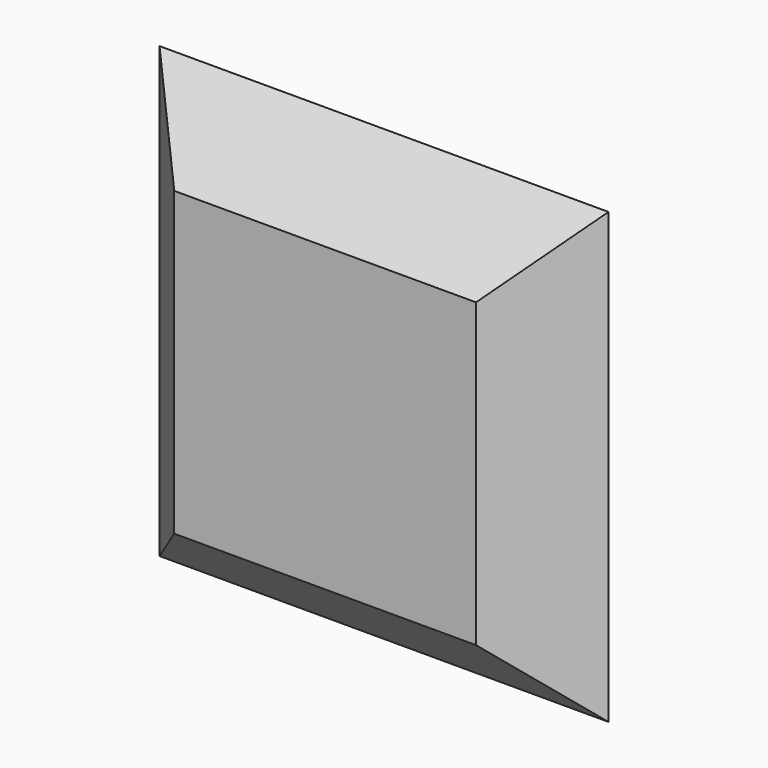
from build123d import *

# Parameters (mm, degrees)
F1_DEPTH     = 3
F2_SIZE2     = 1.49999
F2_SIZE      = 1.49999
F3_W         = 1.7351090792
F3_H         = 1.7351090792
F4_DEPTH     = 0.45
F5_T4_DEPTH  = 3.4702181583
F5_T9_DEPTH  = 3.4702181583
F5_T14_DEPTH = 3.4702181583
F5_T19_DEPTH = 3.4702181583
F6_T1_DEPTH  = 16.5056825173
F6_T3_DEPTH  = 16.5056825173


# Not quite as in the source:
# - a fillet or chamfer that OpenCascade refuses, or shapes differently, is made with other operations: its cross-section is extruded or revolved along the edge and cut away or added
# - a fillet or chamfer is up to 0.001 mm smaller than in the source, because OpenCascade refuses the exact size


with BuildPart() as f1:
    # F0 (on Front) → F1 (new body)
    with BuildSketch(Plane.XZ):
        Polygon((4.575161729, 4.575161729), (0, 4.575161729), (-4.575161729, 4.575161729), (-4.575161729, 0), (-4.575161729, -4.575161729), (0, -4.575161729), (4.575161729, -4.575161729), (4.575161729, 0), align=None)
    extrude(amount=F1_DEPTH)

    # F2 (size 1.5 and 1.5 in the source; OpenCascade refuses exactly that, so slightly less here)
    f2_edges = [f1.edges().sort_by_distance(p)[0] for p in [
        (0, -3, 4.575162),
        (-4.575162, -3, 0),
        (0, -3, -4.575162),
        (4.575162, -3, 0),
        (0, 0, 4.575162),
        (-4.575162, 0, 0),
        (0, 0, -4.575162),
        (4.575162, 0, 0),
    ]]
    chamfer(f2_edges, length=F2_SIZE, length2=F2_SIZE2)

    # F3 (on face) → F4 (cut)
    with BuildSketch(Plane(origin=(0, 0, 0), x_dir=(-1, 0, 0), z_dir=(0, 1, 0))):
        Polygon((0, 1.7351090792), (0, 0), (-1.7351090792, 0), (-1.7351090792, -1.7351090792), (0, -1.7351090792), (1.7351090792, -1.7351090792), (1.7351090792, 0), (1.7351090792, 1.7351090792), align=None)
        with Locations((-0.8675545396, 0.8675545396)):
            Rectangle(F3_W, F3_H)
    extrude(amount=-F4_DEPTH, mode=Mode.SUBTRACT)

    # F5: chamfer of 0.6 on 4 edges, made by hand


with BuildPart() as f5_tool2:
    # F5_s3 → F5_t4 (new body)
    with BuildSketch(Plane.YZ.offset(-1.7351090792)):
        Polygon((0.15, 1.7351090792), (-0.45, 1.1351090792), (-0.45, 1.7351090792), align=None)
    extrude(amount=F5_T4_DEPTH)

    split(bisect_by=Plane.XZ, keep=Keep.TOP)


with BuildPart() as f1_1:
    add(f1.part)

    # F5_t1: union F5_tool2
    add(f5_tool2.part)


with BuildPart() as f5_tool7:
    # F5_s8 → F5_t9 (new body)
    with BuildSketch(Plane.XY.offset(1.7351090792)):
        Polygon((1.7351090792, 0.15), (1.1351090792, -0.45), (1.7351090792, -0.45), align=None)
    extrude(amount=-F5_T9_DEPTH)

    split(bisect_by=Plane.XZ, keep=Keep.TOP)


with BuildPart() as f1_2:
    add(f1_1.part)

    # F5_t6: union F5_tool7
    add(f5_tool7.part)


with BuildPart() as f5_tool12:
    # F5_s13 → F5_t14 (new body)
    with BuildSketch(Plane.YZ.offset(1.7351090792)):
        Polygon((0.15, -1.7351090792), (-0.45, -1.1351090792), (-0.45, -1.7351090792), align=None)
    extrude(amount=-F5_T14_DEPTH)

    split(bisect_by=Plane.XZ, keep=Keep.TOP)


with BuildPart() as f1_3:
    add(f1_2.part)

    # F5_t11: union F5_tool12
    add(f5_tool12.part)


with BuildPart() as f5_tool17:
    # F5_s18 → F5_t19 (new body)
    with BuildSketch(Plane.XY.offset(-1.7351090792)):
        Polygon((-1.7351090792, 0.15), (-1.1351090792, -0.45), (-1.7351090792, -0.45), align=None)
    extrude(amount=F5_T19_DEPTH)

    split(bisect_by=Plane.XZ, keep=Keep.TOP)


with BuildPart() as f1_4:
    add(f1_3.part)

    # F5_t16: union F5_tool17
    add(f5_tool17.part)

    # F6: fillet of radius 5 on 4 edges, made by hand

    # F6_s2 → F6_t1 (cut)
    with BuildSketch(Plane.XY.offset(-8.2528412587)):
        with BuildLine():
            ThreePointArc((4.5396378231, -1.4644660941), (2.917521079, -0.3806023374), (1.0041039171, 0))
            Line((1.0041039171, 0), (3.075171729, 0))
            Line((3.075171729, 0), (4.5396378231, -1.4644660941))
        make_face()
        with BuildLine():
            ThreePointArc((-1.0041039171, 0), (-2.917521079, -0.3806023374), (-4.5396378231, -1.4644660941))
            Line((-4.5396378231, -1.4644660941), (-3.075171729, 0))
            Line((-3.075171729, 0), (-1.0041039171, 0))
        make_face()
    extrude(amount=F6_T1_DEPTH, mode=Mode.SUBTRACT)

    # F6_s4 → F6_t3 (cut)
    with BuildSketch(Plane.YZ.offset(-8.2528412587)):
        with BuildLine():
            ThreePointArc((-1.4644660941, 4.5396378231), (-0.3806023374, 2.917521079), (0, 1.0041039171))
            Line((0, 1.0041039171), (0, 3.075171729))
            Line((0, 3.075171729), (-1.4644660941, 4.5396378231))
        make_face()
        with BuildLine():
            ThreePointArc((0, -1.0041039171), (-0.3806023374, -2.917521079), (-1.4644660941, -4.5396378231))
            Line((-1.4644660941, -4.5396378231), (0, -3.075171729))
            Line((0, -3.075171729), (0, -1.0041039171))
        make_face()
    extrude(amount=F6_T3_DEPTH, mode=Mode.SUBTRACT)


solid = f1_4.part
